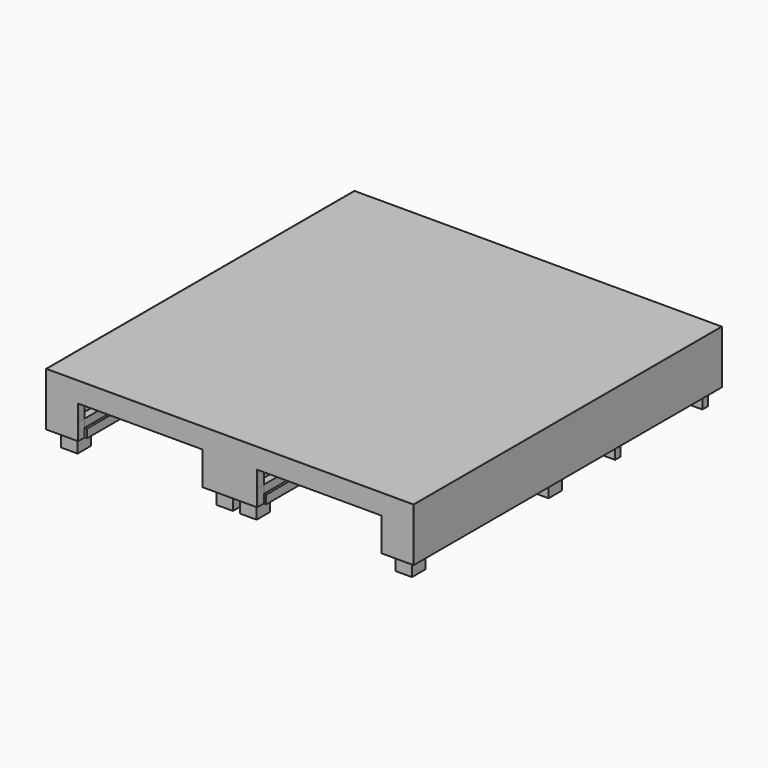
from build123d import *

# Parameters (mm, degrees)
F0_W      = 38.1
F0_H      = 1981.2
F1_DEPTH  = 88.9
F2_W      = 1955.8
F2_H      = 38.1
F3_DEPTH  = 88.9
F4_W      = 958.85
F4_H      = 38.1
F4_W_2    = 38.1
F5_DEPTH  = 88.9
F6_W      = 88.9
F6_H      = 88.9
F7_DEPTH  = 355.6
F6_H_2    = 38.1
F6_H_3    = 37.2039569855
F8_W      = 38.1
F8_H      = 2019.3
F9_DEPTH  = 88.9
F10_W     = 12.7
F10_H     = 45.72
F11_DEPTH = 660.4
F12_W     = 165.1
F12_H     = 88.9
F13_DEPTH = 38.1
F12_W_2   = 292.1
F14_W     = 1955.8
F14_H     = 2057.4
F15_DEPTH = 19.05
F16_W     = 2057.4
F16_H     = 285.75
F17_DEPTH = 6.35
F18_W     = 2057.4
F18_H     = 285.75
F19_DEPTH = 6.35
F20_W     = 292.1
F20_H     = 88.9
F21_DEPTH = 38.1
F20_W_2   = 165.1
F23_DEPTH = 6.35


# Not quite as in the source:
# - a feature names something its author has since deleted; it is built from what else it names


with BuildPart() as f1:
    # F0 (on Top) → F1 (new body)
    with BuildSketch(Plane.XY):
        with Locations((-958.85, 990.6)):
            Rectangle(F0_W, F0_H)
    extrude(amount=F1_DEPTH)


with BuildPart() as f1b:
    # F0 (on Top) → F1, piece 2 (new body)
    with BuildSketch(Plane.XY):
        with Locations((-342.9, 990.6)):
            Rectangle(F0_W, F0_H)
    extrude(amount=F1_DEPTH)


with BuildPart() as f1c:
    # F0 (on Top) → F1, piece 3 (new body)
    with BuildSketch(Plane.XY):
        with Locations((-615.95, 990.6)):
            Rectangle(F0_W, F0_H)
    extrude(amount=F1_DEPTH)


with BuildPart() as f1d:
    # F0 (on Top) → F1, piece 4 (new body)
    with BuildSketch(Plane.XY):
        with Locations((342.9, 990.6)):
            Rectangle(F0_W, F0_H)
    extrude(amount=F1_DEPTH)


with BuildPart() as f1e:
    # F0 (on Top) → F1, piece 5 (new body)
    with BuildSketch(Plane.XY):
        with Locations((615.95, 990.6)):
            Rectangle(F0_W, F0_H)
    extrude(amount=F1_DEPTH)


with BuildPart() as f1f:
    # F0 (on Top) → F1, piece 6 (new body)
    with BuildSketch(Plane.XY):
        with Locations((958.85, 990.6)):
            Rectangle(F0_W, F0_H)
    extrude(amount=F1_DEPTH)


with BuildPart() as f1g:
    # F0 (on Top) → F1, piece 7 (new body)
    with BuildSketch(Plane.XY):
        with Locations((0, 990.6)):
            Rectangle(F0_W, F0_H)
    extrude(amount=F1_DEPTH)


with BuildPart() as f3:
    # F2 (on Top) → F3 (new body)
    with BuildSketch(Plane.XY):
        with Locations((0, 2000.25)):
            Rectangle(F2_W, F2_H)
    extrude(amount=F3_DEPTH)


with BuildPart() as f3b:
    # F2 (on Top) → F3, piece 2 (new body)
    with BuildSketch(Plane.XY):
        with Locations((0, -19.05)):
            Rectangle(F2_W, F2_H)
    extrude(amount=F3_DEPTH)


with BuildPart() as f5:
    # F4 (on face) → F5 (new body)
    with BuildSketch(Plane(origin=(0, 0, 0), x_dir=(1, 0, 0), z_dir=(0, 0, -1))):
        with Locations((-498.475, -1339.85)):
            Rectangle(F4_W, F4_H)
        with Locations((0, -1339.85)):
            Rectangle(F4_W_2, F4_H)
        with Locations((498.475, -1339.85)):
            Rectangle(F4_W, F4_H)
    extrude(amount=F5_DEPTH)


with BuildPart() as f5b:
    # F4 (on face) → F5, piece 2 (new body)
    with BuildSketch(Plane(origin=(0, 0, 0), x_dir=(1, 0, 0), z_dir=(0, 0, -1))):
        with Locations((0, -895.35)):
            Rectangle(F4_W_2, F4_H)
        with Locations((-498.475, -895.35)):
            Rectangle(F4_W, F4_H)
        with Locations((498.475, -895.35)):
            Rectangle(F4_W, F4_H)
    extrude(amount=F5_DEPTH)


with BuildPart() as f7:
    # F6 (on face) → F7 (new body)
    with BuildSketch(Plane.XY.offset(88.9)):
        with Locations((895.35, 44.45)):
            Rectangle(F6_W, F6_H)
    extrude(amount=-F7_DEPTH)


with BuildPart() as f7b:
    # F6 (on face) → F7, piece 2 (new body)
    with BuildSketch(Plane.XY.offset(88.9)):
        with Locations((-895.35, 44.45)):
            Rectangle(F6_W, F6_H)
    extrude(amount=-F7_DEPTH)


with BuildPart() as f7c:
    # F6 (on face) → F7, piece 3 (new body)
    with BuildSketch(Plane.XY.offset(88.9)):
        with Locations((895.35, 958.85)):
            Rectangle(F6_W, F6_H)
    extrude(amount=-F7_DEPTH)


with BuildPart() as f7d:
    # F6 (on face) → F7, piece 4 (new body)
    with BuildSketch(Plane.XY.offset(88.9)):
        with Locations((-895.35, 958.85)):
            Rectangle(F6_W, F6_H)
    extrude(amount=-F7_DEPTH)


with BuildPart() as f7e:
    # F6 (on face) → F7, piece 5 (new body)
    with BuildSketch(Plane.XY.offset(88.9)):
        with Locations((-63.5, 857.25)):
            Rectangle(F6_W, F6_H_2)
    extrude(amount=-F7_DEPTH)


with BuildPart() as f7f:
    # F6 (on face) → F7, piece 6 (new body)
    with BuildSketch(Plane.XY.offset(88.9)):
        with Locations((-63.5, 933.45)):
            Rectangle(F6_W, F6_H_2)
    extrude(amount=-F7_DEPTH)


with BuildPart() as f7g:
    # F6 (on face) → F7, piece 7 (new body)
    with BuildSketch(Plane.XY.offset(88.9)):
        with Locations((63.5, 1301.75)):
            Rectangle(F6_W, F6_H_2)
    extrude(amount=-F7_DEPTH)


with BuildPart() as f7h:
    # F6 (on face) → F7, piece 8 (new body)
    with BuildSketch(Plane.XY.offset(88.9)):
        with Locations((-63.5, 1301.75)):
            Rectangle(F6_W, F6_H_2)
    extrude(amount=-F7_DEPTH)


with BuildPart() as f7i:
    # F6 (on face) → F7, piece 9 (new body)
    with BuildSketch(Plane.XY.offset(88.9)):
        with Locations((63.5, 1377.95)):
            Rectangle(F6_W, F6_H_2)
    extrude(amount=-F7_DEPTH)


with BuildPart() as f7j:
    # F6 (on face) → F7, piece 10 (new body)
    with BuildSketch(Plane.XY.offset(88.9)):
        with Locations((895.35, 1378.3980215073)):
            Rectangle(F6_W, F6_H_3)
    extrude(amount=-F7_DEPTH)


with BuildPart() as f7k:
    # F6 (on face) → F7, piece 11 (new body)
    with BuildSketch(Plane.XY.offset(88.9)):
        with Locations((-895.35, 1377.5019784927)):
            Rectangle(F6_W, F6_H_3)
    extrude(amount=-F7_DEPTH)


with BuildPart() as f7l:
    # F6 (on face) → F7, piece 12 (new body)
    with BuildSketch(Plane.XY.offset(88.9)):
        with Locations((-895.35, 1962.5980215073)):
            Rectangle(F6_W, F6_H_3)
    extrude(amount=-F7_DEPTH)


with BuildPart() as f7m:
    # F6 (on face) → F7, piece 13 (new body)
    with BuildSketch(Plane.XY.offset(88.9)):
        with Locations((895.35, 1962.5980215073)):
            Rectangle(F6_W, F6_H_3)
    extrude(amount=-F7_DEPTH)


with BuildPart() as f7n:
    # F6 (on face) → F7, piece 14 (new body)
    with BuildSketch(Plane.XY.offset(88.9)):
        with Locations((63.5, 44.45)):
            Rectangle(F6_W, F6_H)
    extrude(amount=-F7_DEPTH)


with BuildPart() as f7o:
    # F6 (on face) → F7, piece 15 (new body)
    with BuildSketch(Plane.XY.offset(88.9)):
        with Locations((-63.5, 44.45)):
            Rectangle(F6_W, F6_H)
    extrude(amount=-F7_DEPTH)


with BuildPart() as f7p:
    # F6 (on face) → F7, piece 16 (new body)
    with BuildSketch(Plane.XY.offset(88.9)):
        with Locations((-63.5, 1377.95)):
            Rectangle(F6_W, F6_H_2)
    extrude(amount=-F7_DEPTH)


with BuildPart() as f7q:
    # F6 (on face) → F7, piece 17 (new body)
    with BuildSketch(Plane.XY.offset(88.9)):
        with Locations((63.5, 857.25)):
            Rectangle(F6_W, F6_H_2)
    extrude(amount=-F7_DEPTH)


with BuildPart() as f7r:
    # F6 (on face) → F7, piece 18 (new body)
    with BuildSketch(Plane.XY.offset(88.9)):
        with Locations((63.5, 933.45)):
            Rectangle(F6_W, F6_H_2)
    extrude(amount=-F7_DEPTH)


with BuildPart() as f7s:
    # F6 (on face) → F7, piece 19 (new body)
    with BuildSketch(Plane.XY.offset(88.9)):
        with Locations((63.5, 1962.5980215073)):
            Rectangle(F6_W, F6_H_3)
    extrude(amount=-F7_DEPTH)


with BuildPart() as f7t:
    # F6 (on face) → F7, piece 20 (new body)
    with BuildSketch(Plane.XY.offset(88.9)):
        with Locations((-63.5, 1962.5980215073)):
            Rectangle(F6_W, F6_H_3)
    extrude(amount=-F7_DEPTH)


with BuildPart() as f9:
    # F8 (on face) → F9 (new body)
    with BuildSketch(Plane(origin=(0, 0, -88.9), x_dir=(1, 0, 0), z_dir=(0, 0, -1))):
        with Locations((831.85, -1009.65)):
            Rectangle(F8_W, F8_H)
    extrude(amount=F9_DEPTH)


with BuildPart() as f9b:
    # F8 (on face) → F9, piece 2 (new body)
    with BuildSketch(Plane(origin=(0, 0, -88.9), x_dir=(1, 0, 0), z_dir=(0, 0, -1))):
        with Locations((-831.85, -1009.65)):
            Rectangle(F8_W, F8_H)
    extrude(amount=F9_DEPTH)


with BuildPart() as f9c:
    # F8 (on face) → F9, piece 3 (new body)
    with BuildSketch(Plane(origin=(0, 0, -88.9), x_dir=(1, 0, 0), z_dir=(0, 0, -1))):
        with Locations((127, -1009.65)):
            Rectangle(F8_W, F8_H)
    extrude(amount=F9_DEPTH)


with BuildPart() as f9d:
    # F8 (on face) → F9, piece 4 (new body)
    with BuildSketch(Plane(origin=(0, 0, -88.9), x_dir=(1, 0, 0), z_dir=(0, 0, -1))):
        with Locations((-127, -1009.65)):
            Rectangle(F8_W, F8_H)
    extrude(amount=F9_DEPTH)


with BuildPart() as f9e:
    # F8 (on face) → F9, piece 5 (new body)
    with BuildSketch(Plane(origin=(0, 0, -88.9), x_dir=(1, 0, 0), z_dir=(0, 0, -1))):
        with Locations((958.85, -1009.65)):
            Rectangle(F8_W, F8_H)
    extrude(amount=F9_DEPTH)


with BuildPart() as f9f:
    # F8 (on face) → F9, piece 6 (new body)
    with BuildSketch(Plane(origin=(0, 0, -88.9), x_dir=(1, 0, 0), z_dir=(0, 0, -1))):
        with Locations((-958.85, -1009.65)):
            Rectangle(F8_W, F8_H)
    extrude(amount=F9_DEPTH)


with BuildPart() as f11:
    # F10 (on Front) → F11 (new body)
    with BuildSketch(Plane.XZ):
        with Locations((152.4, -154.94)):
            Rectangle(F10_W, F10_H)
    extrude(amount=-F11_DEPTH)


with BuildPart() as f11b:
    # F10 (on Front) → F11, piece 2 (new body)
    with BuildSketch(Plane.XZ):
        with Locations((-152.4, -154.94)):
            Rectangle(F10_W, F10_H)
    extrude(amount=-F11_DEPTH)


with BuildPart() as f11c:
    # F10 (on Front) → F11, piece 3 (new body)
    with BuildSketch(Plane.XZ):
        with Locations((806.45, -154.94)):
            Rectangle(F10_W, F10_H)
    extrude(amount=-F11_DEPTH)


with BuildPart() as f11d:
    # F10 (on Front) → F11, piece 4 (new body)
    with BuildSketch(Plane.XZ):
        with Locations((-806.45, -154.94)):
            Rectangle(F10_W, F10_H)
    extrude(amount=-F11_DEPTH)


with BuildPart() as f13:
    # F12 (on Front) → F13 (new body)
    with BuildSketch(Plane.XZ):
        with Locations((895.35, -133.35)):
            Rectangle(F12_W, F12_H)
    extrude(amount=F13_DEPTH)


with BuildPart() as f13b:
    # F12 (on Front) → F13, piece 2 (new body)
    with BuildSketch(Plane.XZ):
        with Locations((0, -133.35)):
            Rectangle(F12_W_2, F12_H)
    extrude(amount=F13_DEPTH)


with BuildPart() as f13c:
    # F12 (on Front) → F13, piece 3 (new body)
    with BuildSketch(Plane.XZ):
        with Locations((-895.35, -133.35)):
            Rectangle(F12_W, F12_H)
    extrude(amount=F13_DEPTH)


with BuildPart() as f15:
    # F14 (on face) → F15 (new body)
    with BuildSketch(Plane.XY.offset(88.9)):
        with Locations((0, 990.6)):
            Rectangle(F14_W, F14_H)
    extrude(amount=F15_DEPTH)


with BuildPart() as f17:
    # F16 (on face) → F17 (new body)
    with BuildSketch(Plane.YZ.offset(977.9)):
        with Locations((990.6, -34.925)):
            Rectangle(F16_W, F16_H)
    extrude(amount=F17_DEPTH)


with BuildPart() as f19:
    # F18 (on face) → F19 (new body)
    with BuildSketch(Plane(origin=(-977.9, 0, 0), x_dir=(0, -1, 0), z_dir=(-1, 0, 0))):
        with Locations((-990.6, -34.925)):
            Rectangle(F18_W, F18_H)
    extrude(amount=F19_DEPTH)


with BuildPart() as f21:
    # F20 (on face) → F21 (new body)
    with BuildSketch(Plane.XZ):
        with Locations((0, -44.45)):
            Rectangle(F20_W, F20_H)
    extrude(amount=F21_DEPTH)


with BuildPart() as f21b:
    # F20 (on face) → F21, piece 2 (new body)
    with BuildSketch(Plane.XZ):
        with Locations((895.35, -44.45)):
            Rectangle(F20_W_2, F20_H)
    extrude(amount=F21_DEPTH)


with BuildPart() as f21c:
    # F20 (on face) → F21, piece 3 (new body)
    with BuildSketch(Plane.XZ):
        with Locations((-895.35, -44.45)):
            Rectangle(F20_W_2, F20_H)
    extrude(amount=F21_DEPTH)


with BuildPart() as f23:
    # F22 (on face) → F23 (new body)
    with BuildSketch(Plane.XZ.offset(38.1)):
        Polygon((-984.25, 107.95), (-984.25, -177.8), (-812.8, -177.8), (-812.8, 0), (-146.05, 0), (-146.05, -177.8), (146.05, -177.8), (146.05, 0), (812.8, 0), (812.8, -177.8), (984.25, -177.8), (984.25, 107.95), align=None)
    extrude(amount=F23_DEPTH)


solid = Compound([f1.part, f1b.part, f1c.part, f1d.part, f1e.part, f1f.part, f1g.part, f3.part, f3b.part, f5.part, f5b.part, f7.part, f7b.part, f7c.part, f7d.part, f7e.part, f7f.part, f7g.part, f7h.part, f7i.part, f7j.part, f7k.part, f7l.part, f7m.part, f7n.part, f7o.part, f7p.part, f7q.part, f7r.part, f7s.part, f7t.part, f9.part, f9b.part, f9c.part, f9d.part, f9e.part, f9f.part, f11.part, f11b.part, f11c.part, f11d.part, f13.part, f13b.part, f13c.part, f15.part, f17.part, f19.part, f21.part, f21b.part, f21c.part, f23.part])
